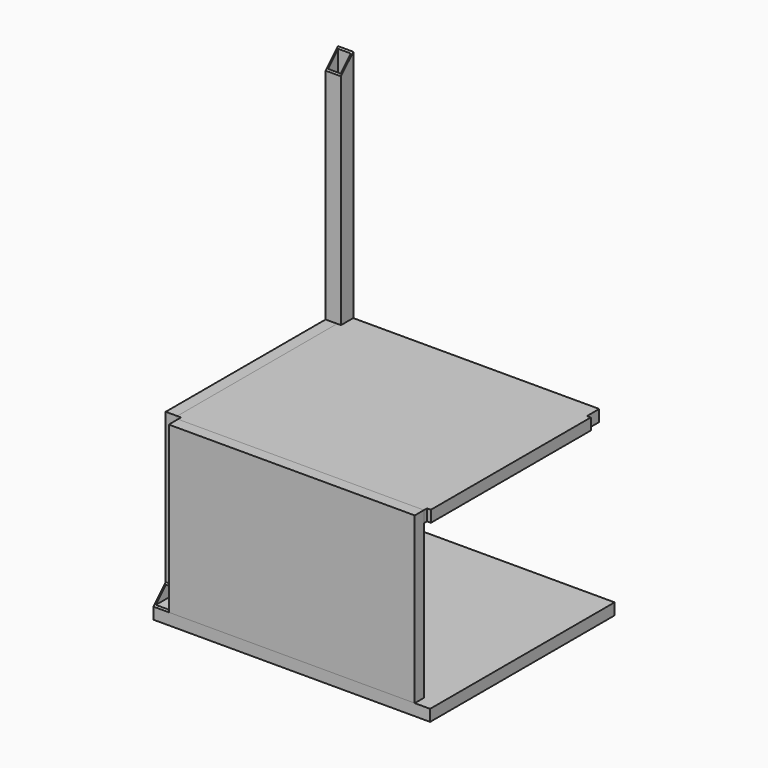
from build123d import *

# Parameters (mm, degrees)
F0_W      = 25.4
F0_H      = 25.4
F0_W_2    = 20.828
F0_H_2    = 20.828
F1_DEPTH  = 660.4
F3_DEPTH  = 25.4
F5_DEPTH  = 25.4
F6_W      = 25.4
F6_H      = 25.4
F6_W_2    = 20.828
F6_H_2    = 20.828
F7_DEPTH  = 381
F9_DEPTH  = 25.4
F10_W     = 457.2
F10_H     = 381
F11_DEPTH = 19.05
F14_DEPTH = 19.05
F15_W     = 330.2
F15_H     = 247.65
F16_DEPTH = 19.05
F17_W     = 406.4
F17_H     = 273.05
F18_DEPTH = 19.05


with BuildPart() as f1:
    # F0 (on Top) → F1 (new body)
    with BuildSketch(Plane.XY):
        with Locations((12.7, -12.7)):
            Rectangle(F0_W, F0_H)
        with Locations((12.7, -12.7)):
            Rectangle(F0_W_2, F0_H_2, mode=Mode.SUBTRACT)
    extrude(amount=F1_DEPTH)

    # F2 (on Right) → F3 (cut)
    with BuildSketch(Plane.YZ):
        Polygon((-25.4, 0), (0, 0), (-25.4, 25.4), align=None)
    extrude(amount=F3_DEPTH, mode=Mode.SUBTRACT)

    # F4 (on face) → F5 (cut, through all)
    with BuildSketch(Plane(origin=(0, 0, 0), x_dir=(0, -1, 0), z_dir=(-1, 0, 0))):
        Polygon((25.4, 660.4), (0, 660.4), (25.4, 635), align=None)
    extrude(amount=-F5_DEPTH, mode=Mode.SUBTRACT)


with BuildPart() as f7:
    # F6 (on Front) → F7 (new body)
    with BuildSketch(Plane.XZ):
        with Locations((12.7, 12.7)):
            Rectangle(F6_W, F6_H)
        with Locations((12.7, 12.7)):
            Rectangle(F6_W_2, F6_H_2, mode=Mode.SUBTRACT)
    extrude(amount=F7_DEPTH)

    # F8 (on face) → F9 (cut, through all)
    with BuildSketch(Plane(origin=(0, 0, 0), x_dir=(0, -1, 0), z_dir=(-1, 0, 0))):
        Polygon((355.6, 25.4), (381, 0), (381, 25.4), align=None)
        Polygon((0, 25.4), (0, 0), (25.4, 25.4), align=None)
    extrude(amount=-F9_DEPTH, mode=Mode.SUBTRACT)


with BuildPart() as f11:
    # F10 (on Top) → F11 (new body)
    with BuildSketch(Plane.XY):
        with Locations((228.6, -190.5)):
            Rectangle(F10_W, F10_H)
    extrude(amount=-F11_DEPTH)


with BuildPart() as f14:
    # F13 (on offset) → F14 (new body)
    with BuildSketch(Plane.XY.offset(254)):
        Polygon((431.8, 0), (25.4, 0), (25.4, -25.4), (19.05, -25.4), (19.05, -355.6), (25.4000000002, -355.6), (25.4, -361.95), (431.8, -361.95), (431.8, -355.6), (438.15, -355.6), (438.15, -25.4), (431.8, -25.4), align=None)
    extrude(amount=F14_DEPTH)


with BuildPart() as f16:
    # F15 (on Right) → F16 (new body)
    with BuildSketch(Plane.YZ):
        with Locations((-190.5, 149.225)):
            Rectangle(F15_W, F15_H)
    extrude(amount=F16_DEPTH)


with BuildPart() as f18:
    # F17 (on face) → F18 (new body)
    with BuildSketch(Plane.XZ.offset(381)):
        with Locations((228.6, 136.525)):
            Rectangle(F17_W, F17_H)
    extrude(amount=-F18_DEPTH)


solid = Compound([f1.part, f7.part, f11.part, f14.part, f16.part, f18.part])
